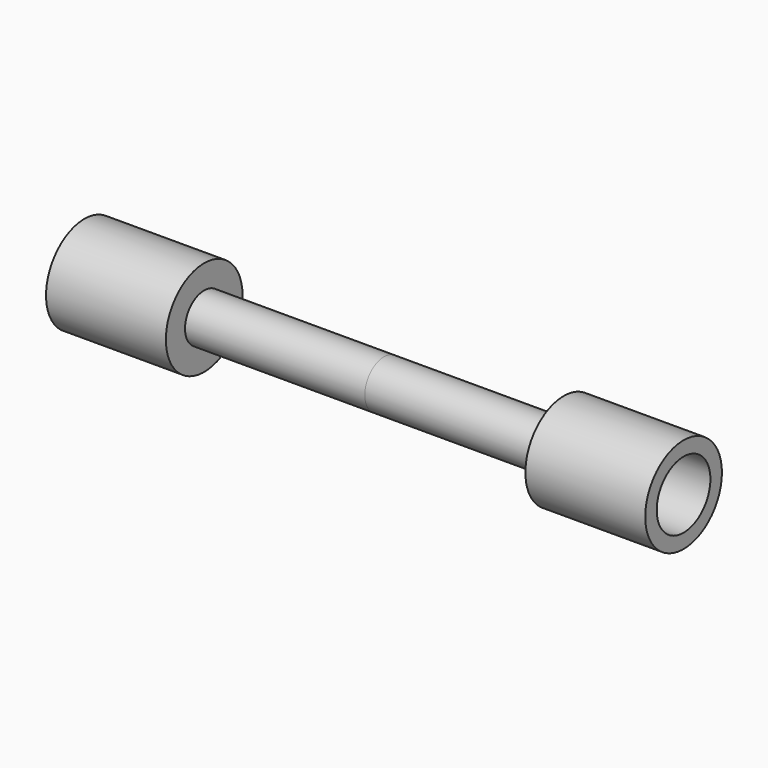
from build123d import *

# Parameters (mm, degrees)
F0_R     = 6
F0_R_2   = 4.2
F1_DEPTH = 12.5
F0_R_3   = 3
F2_DEPTH = 2.5
F3_DEPTH = 25


# Not quite as in the source:
# - a feature names something its author has since deleted; it is built from what else it names


with BuildPart() as f1:
    # F0 (on Right) → F1 (new body)
    with BuildSketch(Plane.YZ):
        Circle(F0_R)
        Circle(F0_R_2, mode=Mode.SUBTRACT)
    extrude(amount=F1_DEPTH)

    # F0 (on Right) → F2 (join)
    with BuildSketch(Plane.YZ):
        Circle(F0_R)
        Circle(F0_R_2, mode=Mode.SUBTRACT)
        Circle(F0_R_2)
        Circle(F0_R_3, mode=Mode.SUBTRACT)
    extrude(amount=-F2_DEPTH)

    # F0 (on Right) → F3 (join)
    with BuildSketch(Plane.YZ):
        Circle(F0_R_3)
    extrude(amount=-F3_DEPTH)


with BuildPart() as f4_1:
    # F4: instance of F1
    add(f1.part.mirror(Plane(origin=(-25, 0, 0), x_dir=(0, 1, 0), z_dir=(-1, 0, 0))))


solid = Compound([f1.part, f4_1.part])
